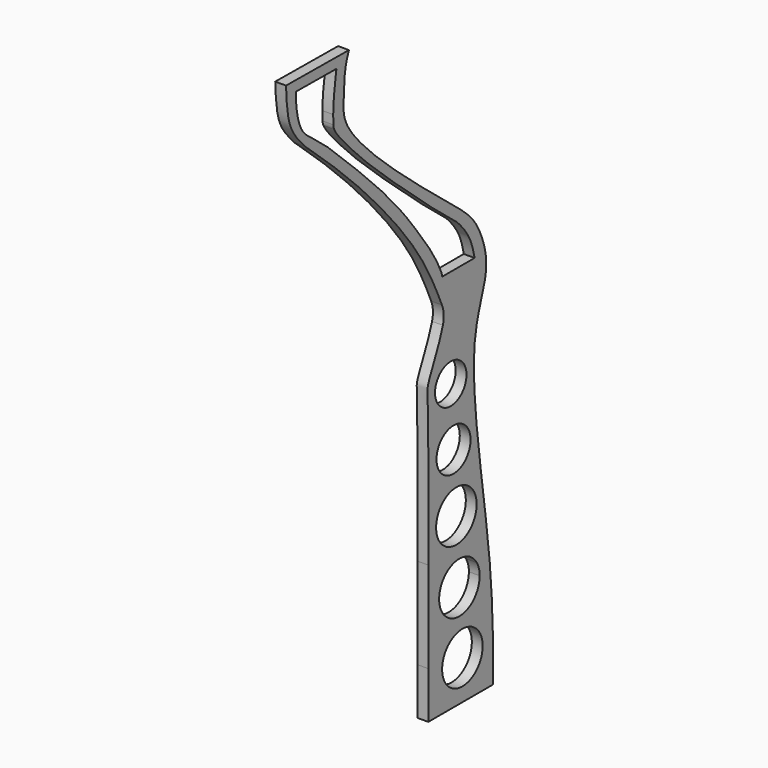
from build123d import *

# Parameters (mm, degrees)
F0_R     = 4.6883037194
F0_R_2   = 3.9392661415
F0_R_3   = 3.6384688305
F1_DEPTH = 2


with BuildPart() as f1:
    # F0 (on Right) → F1 (new body)
    with BuildSketch(Plane.YZ):
        with BuildLine():
            ThreePointArc((79.8957550101, 17.6550047898), (80.2951283262, 15.98002463), (80.1025933871, 14.268888201))
            add(Edge.make_bspline(
                [(80.4956108332, 16.2556357682), (80.4570591964, 15.6645429926), (80.3133675624, 14.9880382733), (80.1025933871, 14.268888201)],
                knots=[0.1450341549, 0.1450341549, 0.1450341549, 0.1450341549, 0.1920697624, 0.1920697624, 0.1920697624, 0.1920697624], degree=3))
            add(Edge.make_bspline(
                [(79.8957550101, 17.6550047898), (80.0971506674, 17.1879589655), (80.2963799136, 16.7218081376), (80.4956108332, 16.2556357682)],
                knots=[0.9662359683, 0.9662359683, 0.9662359683, 0.9662359683, 1, 1, 1, 1], degree=3))
        make_face()
        with BuildLine():
            add(Edge.make_bspline(
                [(80.1025933871, 14.268888201), (79.2865163427, 11.4844775171), (76.3746678901, 6.0119629795), (76.7192801107, 4.392209), (76.7670835041, -9.947638286), (76.7624697083, -23.4316956947)],
                knots=[0.1920697624, 0.1920697624, 0.1920697624, 0.1920697624, 0.3741825829, 0.4831625245, 0.8093358927, 0.8093358927, 0.8093358927, 0.8093358927], degree=3))
            add(Edge.make_bspline(
                [(76.7624697083, -23.4316956947), (78.7015422133, -24.1477778796), (80.6205636372, -24.8568445533), (82.4325372304, -25.5284571248)],
                knots=[0.0270811096, 0.0270811096, 0.0270811096, 0.0270811096, 0.1445794371, 0.1445794371, 0.1445794371, 0.1445794371], degree=3))
            ThreePointArc((82.4325372304, -25.5284571248), (85.5593685519, -25.5804488455), (87.957885412, -27.5871611128))
            add(Edge.make_bspline(
                [(87.957885412, -27.5871611128), (89.0859034651, -28.0107819184), (90.0933921461, -28.3922316739), (90.9407654034, -28.7176599349)],
                knots=[0.2751664288, 0.2751664288, 0.2751664288, 0.2751664288, 0.3655406854, 0.3655406854, 0.3655406854, 0.3655406854], degree=3))
            add(Edge.make_bspline(
                [(57.1466498224, 58.7420705596), (57.1602811091, 57.8399433674), (58.5817092979, 51.97360927), (82.8041301063, 32.7009203844), (88.0099023997, 28.3107089105), (91.5680094157, 18.9712767827), (84.7466815595, 8.6428960087), (89.5974882958, -15.9942043752), (90.8703512806, -28.0068250998), (90.9407654034, -28.7176599349)],
                knots=[0.0416229957, 0.0416229957, 0.0416229957, 0.0416229957, 0.0848091888, 0.2906596564, 0.3924191098, 0.4932200917, 0.6135562047, 0.8271488441, 0.8408588658, 0.8408588658, 0.8408588658, 0.8408588658], degree=3))
            Line((57.1466498224, 58.7420705596), (57.12578985, 59.5825674036))
            add(Edge.make_bspline(
                [(57.12578985, 59.5825674036), (57.1896981946, 61.6323841738), (57.2990368452, 65.1393471722), (58.0594427733, 67.1134882981), (58.3753921092, 67.9337456822)],
                knots=[0, 0, 0, 0, 0.5844991154, 1, 1, 1, 1], degree=3))
            Line((58.3753921092, 67.9337456822), (43.8300706446, 68.0636242032))
            add(Edge.make_bspline(
                [(48.1593688821, 56.4218290004), (46.8770978389, 57.7977564654), (44.1432493691, 60.7312838303), (43.9386863932, 65.5206429075), (43.8300706446, 68.0636242032)],
                knots=[0, 0, 0, 0, 0.4690351559, 1, 1, 1, 1], degree=3))
            Line((48.1593688821, 56.4218290004), (49.8435108373, 54.9144878378))
            add(Edge.make_bspline(
                [(49.8435108373, 54.9144878378), (52.815529184, 52.2776531088), (61.4394394987, 44.3447683348), (74.484501975, 29.6593432966), (78.4365909399, 21.0388736118), (79.8957550101, 17.6550047898)],
                knots=[0.154333465, 0.154333465, 0.154333465, 0.154333465, 0.3515724353, 0.7216067518, 0.9662359683, 0.9662359683, 0.9662359683, 0.9662359683], degree=3))
            add(Edge.make_bspline(
                [(79.8957550101, 17.6550047898), (80.0971506674, 17.1879589655), (80.2963799136, 16.7218081376), (80.4956108332, 16.2556357682)],
                knots=[0.9662359683, 0.9662359683, 0.9662359683, 0.9662359683, 1, 1, 1, 1], degree=3))
            add(Edge.make_bspline(
                [(80.4956108332, 16.2556357682), (80.4570591964, 15.6645429926), (80.3133675624, 14.9880382733), (80.1025933871, 14.268888201)],
                knots=[0.1450341549, 0.1450341549, 0.1450341549, 0.1450341549, 0.1920697624, 0.1920697624, 0.1920697624, 0.1920697624], degree=3))
        make_face()
        with Locations((83.2207022909, -18.0455071758)):
            Circle(F0_R, mode=Mode.SUBTRACT)
        with Locations((82.568819048, -6.9652261674)):
            Circle(F0_R_2, mode=Mode.SUBTRACT)
        with Locations((81.9228366017, 4.0147569962)):
            Circle(F0_R_3, mode=Mode.SUBTRACT)
        with BuildLine():
            ThreePointArc((54.7713492842, 57.2177769689), (54.8271979257, 56.810114984), (54.9652899831, 56.4225095809))
            add(Edge.make_bspline(
                [(54.9652899831, 56.4225095809), (55.4703755244, 55.3642297227), (58.2066489083, 52.3391222765), (63.4153535343, 46.7086525336), (80.6301039509, 31.6847612882), (83.2731553162, 30.0467828266), (86.5691865953, 26.1532190516), (87.1495435558, 23.5312600221), (87.43044734, 22.2621820867)],
                knots=[0.1022523883, 0.1022523883, 0.1022523883, 0.1022523883, 0.2113924531, 0.3848424985, 0.6556235338, 0.7622790828, 0.8849385641, 1, 1, 1, 1], degree=3))
            Line((87.43044734, 22.2621820867), (80.8183178306, 22.2621820867))
            Line((80.8183178306, 22.2621820867), (79.9628868699, 22.2621820867))
            add(Edge.make_bspline(
                [(76.995678246, 28.0477926135), (77.5112858693, 27.2563115148), (78.5327821075, 25.6882684365), (79.7936114735, 23.0629855626), (79.9199958873, 22.4650895896), (79.9628868699, 22.2621820867)],
                knots=[0, 0, 0, 0, 0.4023866175, 0.7971883997, 1, 1, 1, 1], degree=3))
            add(Edge.make_bspline(
                [(53.4740150752, 54.1077444553), (59.0371788567, 48.8936546263), (69.2228621791, 39.0679619057), (74.4568134712, 31.6473528485), (76.995678246, 28.0477926135)],
                knots=[0.1414781195, 0.1414781195, 0.1414781195, 0.1414781195, 0.5835515389, 1, 1, 1, 1], degree=3))
            Line((53.4740150752, 54.1077444553), (49.5728808967, 57.2913064097))
            add(Edge.make_bspline(
                [(49.5728808967, 57.2913064097), (48.7155941015, 57.8834306969), (46.6881680975, 59.6656337099), (46.102100063, 64.4285146744), (46.0896684812, 65.6893778461), (46.0855774581, 66.1456882954)],
                knots=[0.1388258208, 0.1388258208, 0.1388258208, 0.1388258208, 0.382893267, 0.7768741592, 1, 1, 1, 1], degree=3))
            Line((46.0855774581, 66.1456882954), (55.5281094919, 66.0613737549))
            Line((55.5281094919, 66.0613737549), (55.418305099, 65.7329410315))
            add(Edge.make_bspline(
                [(54.7404844243, 58.9079639922), (54.7423727181, 59.352678995), (54.7938891269, 61.3267690629), (55.1474991661, 63.8220073533), (55.418305099, 65.7329410315)],
                knots=[0.2716046575, 0.2716046575, 0.2716046575, 0.2716046575, 0.4421714365, 1, 1, 1, 1], degree=3))
            add(Edge.make_bspline(
                [(54.7713492842, 57.2177769689), (54.7531461092, 57.7675184991), (54.7379986333, 58.3225314814), (54.7404844243, 58.9079639922)],
                knots=[0.0470668364, 0.0470668364, 0.0470668364, 0.0470668364, 0.2716046575, 0.2716046575, 0.2716046575, 0.2716046575], degree=3))
        make_face(mode=Mode.SUBTRACT)
        with BuildLine():
            add(Edge.make_bspline(
                [(76.7624697083, -23.4316956947), (78.7015422133, -24.1477778796), (80.6205636372, -24.8568445533), (82.4325372304, -25.5284571248)],
                knots=[0.0270811096, 0.0270811096, 0.0270811096, 0.0270811096, 0.1445794371, 0.1445794371, 0.1445794371, 0.1445794371], degree=3))
            add(Edge.make_bspline(
                [(76.7624697083, -23.4316956947), (76.7606596316, -28.7217388563), (76.7526244709, -34.4328108048), (76.7425421777, -40.2823389925)],
                knots=[0.8093358927, 0.8093358927, 0.8093358927, 0.8093358927, 0.9372996905, 0.9372996905, 0.9372996905, 0.9372996905], degree=3))
            add(Edge.make_bspline(
                [(76.7425421777, -40.2823389925), (76.7376020078, -43.1485186013), (76.732170352, -46.0479394839), (76.7267386962, -48.9473603666)],
                knots=[0.9372996905, 0.9372996905, 0.9372996905, 0.9372996905, 1, 1, 1, 1], degree=3))
            Line((76.7267386962, -48.9473603666), (91.6395902509, -48.9473603666))
            Line((91.6395902509, -48.9473603666), (91.6395902509, -40.2823389925))
            add(Edge.make_bspline(
                [(90.9407654034, -28.7176599349), (91.3630937503, -32.981090182), (91.5566289372, -36.7509584482), (91.6395902509, -40.2823389925)],
                knots=[0.8408588658, 0.8408588658, 0.8408588658, 0.8408588658, 0.9230885456, 0.9230885456, 0.9230885456, 0.9230885456], degree=3))
            add(Edge.make_bspline(
                [(87.957885412, -27.5871611128), (89.0859034651, -28.0107819184), (90.0933921461, -28.3922316739), (90.9407654034, -28.7176599349)],
                knots=[0.2751664288, 0.2751664288, 0.2751664288, 0.2751664288, 0.3655406854, 0.3655406854, 0.3655406854, 0.3655406854], degree=3))
            ThreePointArc((87.957885412, -27.5871611128), (88.4446078172, -28.7365892089), (88.6107749153, -29.9737117344))
            ThreePointArc((88.6107749153, -29.9737117344), (81.1843213813, -33.7793296026), (82.4325372304, -25.5284571248))
        make_face()
        with Locations((84.6114576106, -41.6846479636)):
            Circle(F0_R, mode=Mode.SUBTRACT)
    extrude(amount=F1_DEPTH)


solid = f1.part
